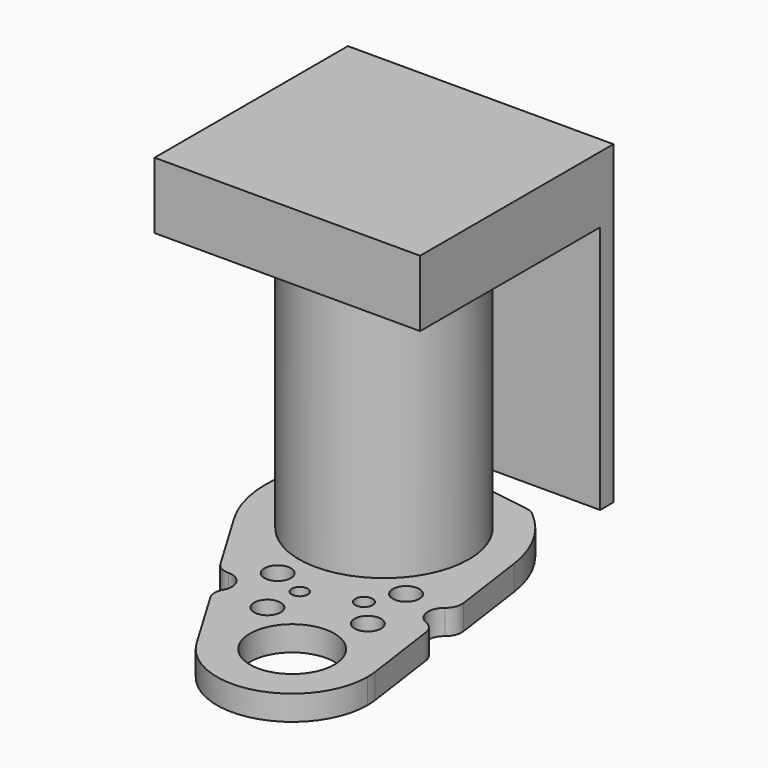
from build123d import *

# Parameters (mm, degrees)
F0_W      = 101.6
F0_H      = 152.4
F1_DEPTH  = 9.525
F2_R      = 32.512
F2_R_2    = 16.129
F3_DEPTH  = 25.4
F5_DEPTH  = 25.4
F6_R      = 33.02
F6_R_2    = 24.13
F7_DEPTH  = 6.35
F9_DEPTH  = 25.4
F10_R     = 1.905
F11_DEPTH = 25.4
F12_R     = 5.08
F13_DEPTH = 6.985
F14_R     = 3.302
F14_R_2   = 3.048
F15_DEPTH = 25.4
F16_R     = 32.4993
F17_DEPTH = 101.6
F18_W     = 101.6
F18_H     = 92.456
F19_DEPTH = 25.4
F20_W     = 101.6
F20_H     = 6.35
F21_DEPTH = 95.25
F22_R     = 6.35
F23_R     = 2.032


with BuildPart() as f1:
    # F0 (on Top) → F1 (new body)
    with BuildSketch(Plane.XY):
        with Locations((50.8, 76.2)):
            Rectangle(F0_W, F0_H)
    extrude(amount=F1_DEPTH)

    # F2 (on face) → F3 (cut)
    with BuildSketch(Plane.XY.offset(9.525)):
        with Locations((45.212, 107.188)):
            Circle(F2_R)
        with Locations((72.771, 28.829)):
            Circle(F2_R_2)
    extrude(amount=-F3_DEPTH, mode=Mode.SUBTRACT)

    # F4 (on face) → F5 (cut)
    with BuildSketch(Plane.XY.offset(9.525)):
        with BuildLine():
            Line((0, 0), (72.7710000733, 0))
            ThreePointArc((72.7710000733, 0), (58.5206703615, 3.768286798), (47.9957095185, 14.0880291175))
            Line((47.9957095185, 14.0880291175), (30.4234443558, 43.6219029237))
            ThreePointArc((30.4234443558, 43.6219029237), (32.6336469107, 52.3259252506), (23.9296245838, 54.5361278054))
            Line((23.9296245838, 54.5361278054), (6.3573594211, 84.0700016116))
            ThreePointArc((6.3573594211, 84.0700016116), (1.6183023256, 95.1999031088), (0, 107.188))
            Line((0, 107.188), (0, 0))
        make_face()
        with BuildLine():
            Line((7.2246134342, 131.7050023841), (0, 138.9296158184))
            Line((0, 138.9296158184), (0, 107.188))
            ThreePointArc((0, 107.188), (1.8437474101, 119.9676561493), (7.2246134342, 131.7050023841))
        make_face()
        Polygon((0, 138.9296158184), (13.4703841816, 152.4), (0, 152.4), align=None)
        with BuildLine():
            ThreePointArc((72.4437617696, 143.2789420066), (84.1747986467, 130.1232406923), (89.9838196578, 113.4815767678))
            Line((89.9838196578, 113.4815767678), (94.7676421119, 79.4499848615))
            ThreePointArc((94.7676421119, 79.4499848615), (89.363394515, 72.277878622), (96.5355007546, 66.8736310251))
            Line((96.5355007546, 66.8736310251), (101.3193232087, 32.8420391188))
            ThreePointArc((101.3193232087, 32.8420391188), (101.5297452052, 30.8404211947), (101.6, 28.8289998081))
            Line((101.6, 28.8289998081), (101.6, 152.4))
            Line((101.6, 152.4), (13.4703841816, 152.4))
            Line((13.4703841816, 152.4), (20.6949976159, 145.1753865658))
            ThreePointArc((20.6949976159, 145.1753865658), (25.3824997549, 147.8194639661), (30.3509720516, 149.8878219237))
            Line((30.3509720516, 149.8878219237), (72.4437617696, 143.2789420066))
        make_face()
        with BuildLine():
            Line((101.6, 0), (101.6, 28.8289998081))
            ThreePointArc((101.6, 28.8289998081), (93.1561813529, 8.4438185632), (72.7710000733, 0))
            Line((72.7710000733, 0), (101.6, 0))
        make_face()
    extrude(amount=-F5_DEPTH, mode=Mode.SUBTRACT)

    # F6 (on face) → F7 (join)
    with BuildSketch(Plane(origin=(0, 0, 0), x_dir=(1, 0, 0), z_dir=(0, 0, -1))):
        with Locations((45.212, -107.188)):
            Circle(F6_R)
        with Locations((45.212, -107.188)):
            Circle(F6_R_2, mode=Mode.SUBTRACT)
    extrude(amount=-F7_DEPTH)

    # F8 (on face) → F9 (cut)
    with BuildSketch(Plane.XY.offset(9.525)):
        Polygon((29.6315491221, 124.5645021021), (7.6332177029, 146.5628335213), (5.8371664787, 144.7667822971), (27.8354978979, 122.7684508779), align=None)
    extrude(amount=-F9_DEPTH, mode=Mode.SUBTRACT)

    # F10 (on face) → F11 (cut)
    with BuildSketch(Plane(origin=(69.4648079092, 69.4648079092, 0), x_dir=(0.7071067812, -0.7071067812, 0), z_dir=(-0.7071067812, -0.7071067812, 0))):
        with Locations((-93.129500302, 4.7625)):
            Circle(F10_R)
    extrude(amount=-F11_DEPTH, mode=Mode.SUBTRACT)

    # F12 (on face) → F13 (cut)
    with BuildSketch(Plane.XY.offset(9.525)):
        with Locations((38.6882198833, 64.5036622051)):
            Circle(F12_R)
        with Locations((77.0188242242, 77.9846040883)):
            Circle(F12_R)
        with Locations((80.1401720853, 55.7796753677)):
            Circle(F12_R)
        with Locations((50.1537692021, 45.2334040134)):
            Circle(F12_R)
    extrude(amount=-F13_DEPTH, mode=Mode.SUBTRACT)

    # F14 (on face) → F15 (cut)
    with BuildSketch(Plane.XY.offset(9.525)):
        with Locations((70.4493668127, 66.0528214254)):
            Circle(F14_R)
        with Locations((51.2803585402, 59.3110470411)):
            Circle(F14_R_2)
    extrude(amount=-F15_DEPTH, mode=Mode.SUBTRACT)

    # F22
    f22_edges = [f1.edges().sort_by_distance(p)[0] for p in [
        (94.767642, 79.449985, 4.7625),
        (96.535501, 66.873631, 4.7625),
        (23.929625, 54.536128, 4.7625),
        (30.423444, 43.621903, 4.7625),
        (72.443762, 143.278942, 4.7625),
        (30.350972, 149.887822, 4.7625),
    ]]
    fillet(f22_edges, radius=F22_R)

    # F23
    f23_edges = [f1.edges().sort_by_distance(p)[0] for p in [
        (7.633218, 146.562834, 4.7625),
        (5.837166, 144.766782, 4.7625),
        (7.224613, 131.705002, 4.7625),
        (20.694998, 145.175387, 4.7625),
        (27.275136, 123.328812, 3.175),
        (29.071188, 125.124864, 3.175),
        (0, 138.929616, 4.7625),
        (13.470384, 152.4, 4.7625),
    ]]
    fillet(f23_edges, radius=F23_R)


with BuildPart() as f17:
    # F16 (on face) → F17 (new body)
    with BuildSketch(Plane.XY.offset(9.525)):
        with Locations((45.212, 107.188)):
            Circle(F16_R)
    extrude(amount=F17_DEPTH)

    # F18 (on face) → F19 (join)
    with BuildSketch(Plane.XY.offset(111.125)):
        with Locations((45.212, 107.188)):
            Rectangle(F18_W, F18_H)
    extrude(amount=F19_DEPTH)

    # F20 (on face) → F21 (join)
    with BuildSketch(Plane(origin=(0, 0, 111.125), x_dir=(1, 0, 0), z_dir=(0, 0, -1))):
        with Locations((45.212, -150.241)):
            Rectangle(F20_W, F20_H)
    extrude(amount=F21_DEPTH)


solid = Compound([f1.part, f17.part])
